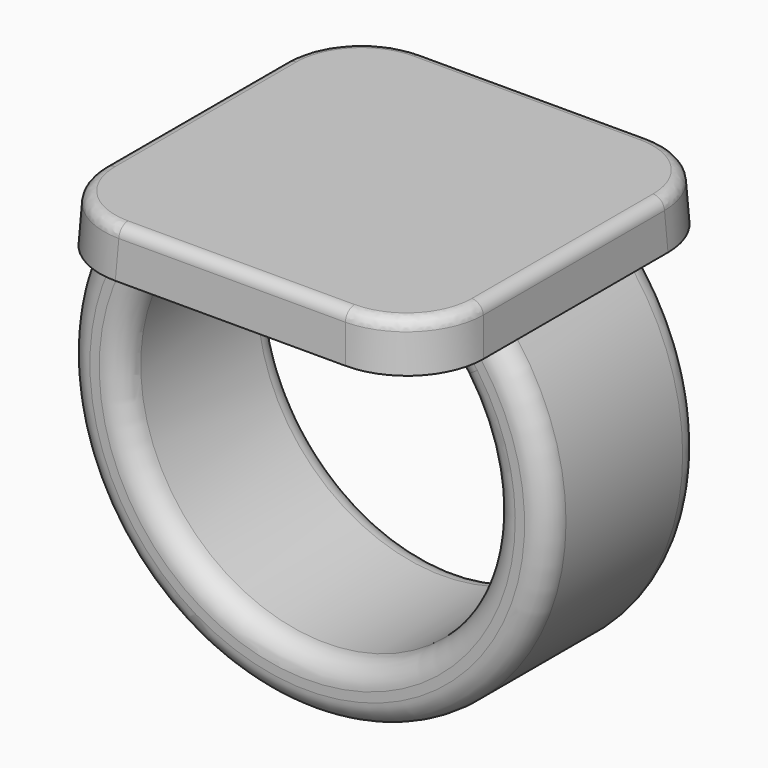
from build123d import *

# Parameters (mm, degrees)
F0_W          = 25.4
F0_H          = 25.4
F1_DEPTH      = 3.175
F1_TAPER      = 3
F3_W          = 5.08
F3_H          = 12.7
F6_DEPTH      = 6.35
F6_DEPTH_BACK = 6.35
F7_R          = 5.08
F8_R          = 1.524
F9_R          = 0.762


with BuildPart() as f1:
    # F0 (on Top) → F1 (new body)
    with BuildSketch(Plane.XY):
        Rectangle(F0_W, F0_H)
    extrude(amount=F1_DEPTH, taper=F1_TAPER)

    # F4: sweep along a path in F2
    with BuildLine(Plane.XZ) as f4_path:
        ThreePointArc((-10.16, 0), (0, -23.5582897328), (10.16, 0))
    # F3 (on face) → F4 (sweep)
    with BuildSketch(Plane(origin=(0, 0, 0), x_dir=(1, 0, 0), z_dir=(0, 0, -1))):
        with Locations((-10.16, 0)):
            Rectangle(F3_W, F3_H)
    sweep(path=f4_path.line)

    # F5 (on Front) → F6 (join, two sides)
    with BuildSketch(Plane.XZ) as f6_sk:
        with BuildLine():
            Line((10.0130578512, -2.535746045), (10.16, 0))
            Line((10.16, 0), (7.62, 0))
            ThreePointArc((7.62, 0), (8.9072265211, -1.1822790439), (10.0130578512, -2.535746045))
        make_face()
    extrude(amount=F6_DEPTH)
    extrude(f6_sk.sketch, amount=-F6_DEPTH_BACK)

    # F7
    f7_edges = [f1.edges().sort_by_distance(p)[0] for p in [
        (-12.616803, 12.616803, 1.5875),
        (12.616803, 12.616803, 1.5875),
        (12.616803, -12.616803, 1.5875),
        (-12.616803, -12.616803, 1.5875),
    ]]
    fillet(f7_edges, radius=F7_R)

    # F8
    f8_edges = [f1.edges().sort_by_distance(p)[0] for p in [
        (-1.743325, -6.35, -21.711017),
        (8.907227, -6.35, -1.182279),
        (-1.743325, 6.35, -21.711017),
        (0, -6.35, -25.501344),
        (0, 6.35, -25.501344),
        (8.907227, 6.35, -1.182279),
    ]]
    fillet(f8_edges, radius=F8_R)

    # F9
    f9_edges = [f1.edges().sort_by_distance(p)[0] for p in [
        (12.533605, 0, 3.175),
        (11.048589, -11.048589, 3.175),
        (11.048589, 11.048589, 3.175),
        (0, -12.533605, 3.175),
        (0, 12.533605, 3.175),
        (-11.048589, -11.048589, 3.175),
        (-11.048589, 11.048589, 3.175),
        (-12.533605, 0, 3.175),
    ]]
    fillet(f9_edges, radius=F9_R)


solid = f1.part
